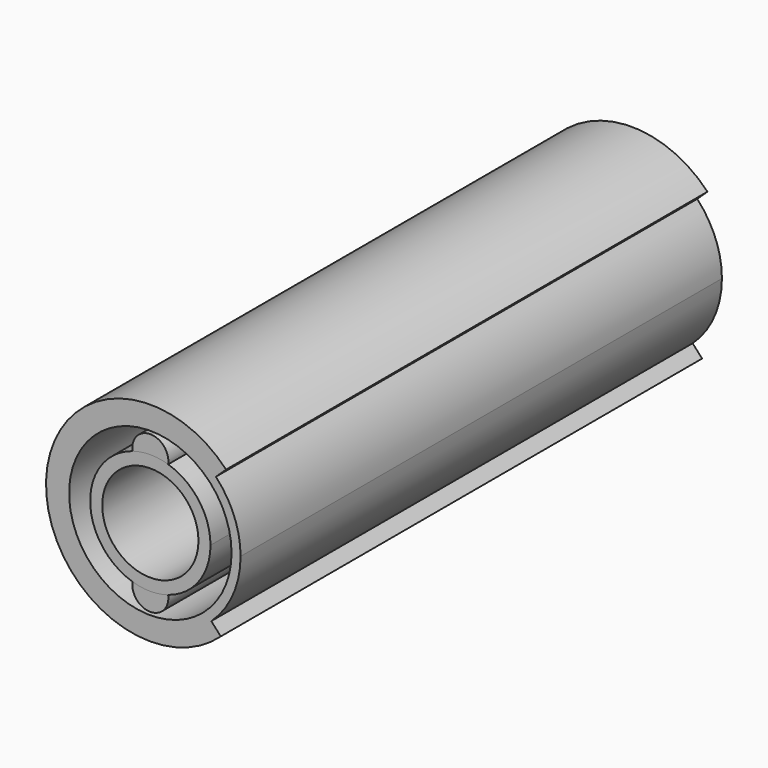
from build123d import *

# Parameters (mm, degrees)
F8_DEPTH  = 63.5
F9_DEPTH  = 63.5
F10_DEPTH = 63.5
F0_R      = 17.145
F11_DEPTH = 63.5
F0_R_2    = 10.16
F12_DEPTH = 63.5


# Not quite as in the source:
# - the program builds the solid bodies; features that only make, move or delete a surface that nothing else refers to are left out


with BuildPart() as f8:
    # F0 (on Front) → F8 (new body, symmetric)
    with BuildSketch(Plane.XZ):
        with BuildLine():
            ThreePointArc((12.8668441558, -14.0480184179), (-19.037832377, 0.6807630905), (13.8373687009, 13.0931175598))
            Line((13.8373687009, 13.0931175598), (15.9931019877, 15.1329034441))
            ThreePointArc((15.9931019877, 15.1329034441), (-22.0037495142, 0.7868196455), (14.8713787493, -16.2365689705))
            Line((14.8713787493, -16.2365689705), (12.8668441558, -14.0480184179))
        make_face()
    extrude(amount=F8_DEPTH, both=True)

    # F0 (on Front) → F11 (join, symmetric)
    with BuildSketch(Plane.XZ):
        with BuildLine():
            ThreePointArc((12.8668441558, -14.0480184179), (17.4358234845, -7.6742790812), (19.05, 0))
            ThreePointArc((19.05, 0), (17.6989318004, 7.0462978311), (13.8373687009, 13.0931175598))
            ThreePointArc((13.8373687009, 13.0931175598), (-19.037832377, 0.6807630905), (12.8668441558, -14.0480184179))
        make_face()
        Circle(F0_R, mode=Mode.SUBTRACT)
    extrude(amount=F11_DEPTH, both=True)


with BuildPart() as f9:
    # F0 (on Front) → F9 (new body, symmetric)
    with BuildSketch(Plane.XZ):
        with BuildLine():
            ThreePointArc((-3.7668936473, 12.1285), (-1.905, 12.5563121576), (0, 12.7))
            Line((0, 12.7), (0, 16.51))
            ThreePointArc((0, 16.51), (-2.8890755442, 15.1838161164), (-3.7668936473, 12.1285))
        make_face()
    extrude(amount=F9_DEPTH, both=True)

    # F0 (on Front) → F10 (join, symmetric)
    with BuildSketch(Plane.XZ):
        with BuildLine():
            ThreePointArc((0, 12.7), (1.905, 12.5563121576), (3.7668936473, 12.1285))
            ThreePointArc((3.7668936473, 12.1285), (2.8890755442, 15.1838161164), (0, 16.51))
            Line((0, 16.51), (0, 12.7))
        make_face()
    extrude(amount=F10_DEPTH, both=True)


with BuildPart() as f10:
    # F0 (on Front) → F10, piece 2 (new body, symmetric)
    with BuildSketch(Plane.XZ):
        with BuildLine():
            Line((0, -16.51), (0, -12.7))
            ThreePointArc((0, -12.7), (-1.905, -12.5563121576), (-3.7668936473, -12.1285))
            ThreePointArc((-3.7668936473, -12.1285), (-2.8890755442, -15.1838161164), (0, -16.51))
        make_face()
        with BuildLine():
            ThreePointArc((0, -16.51), (2.8890755442, -15.1838161164), (3.7668936473, -12.1285))
            ThreePointArc((3.7668936473, -12.1285), (1.905, -12.5563121576), (0, -12.7))
            Line((0, -12.7), (0, -16.51))
        make_face()
    extrude(amount=F10_DEPTH, both=True)


with BuildPart() as f12:
    # F0 (on Front) → F12 (new body, symmetric)
    with BuildSketch(Plane.XZ):
        with BuildLine():
            ThreePointArc((3.7668936473, -12.1285), (10.2256918915, -7.5316150552), (12.7, 0))
            ThreePointArc((12.7, 0), (10.2256918915, 7.5316150552), (3.7668936473, 12.1285))
            ThreePointArc((3.7668936473, 12.1285), (1.905, 12.5563121576), (0, 12.7))
            ThreePointArc((0, 12.7), (-1.905, 12.5563121576), (-3.7668936473, 12.1285))
            ThreePointArc((-3.7668936473, 12.1285), (-12.7, 0), (-3.7668936473, -12.1285))
            ThreePointArc((-3.7668936473, -12.1285), (-1.905, -12.5563121576), (0, -12.7))
            ThreePointArc((0, -12.7), (1.905, -12.5563121576), (3.7668936473, -12.1285))
        make_face()
        Circle(F0_R_2, mode=Mode.SUBTRACT)
    extrude(amount=F12_DEPTH, both=True)


solid = Compound([f8.part, f9.part, f10.part, f12.part])
